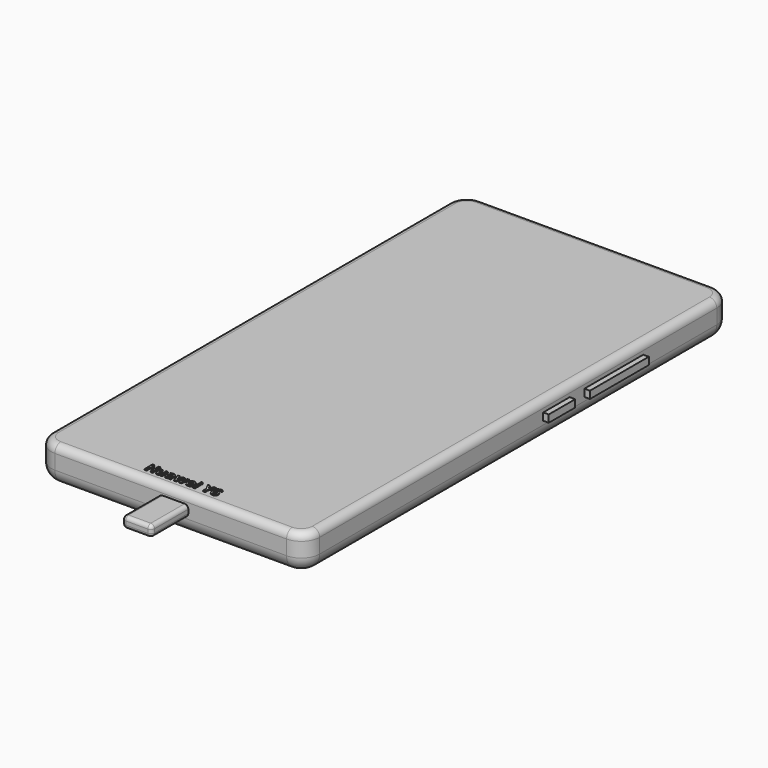
from build123d import *

# Parameters (mm, degrees)
F1_DEPTH      = 10
F2_R          = 2
F3_R          = 4
F4_W          = 20
F4_H          = 2
F5_DEPTH      = 38
F6_W          = 9
F6_H          = 2
F7_DEPTH      = 38
F8_W          = 8
F8_H          = 3
F9_DEPTH      = 85
F10_R         = 1
F11_TEXT_SIZE = 3.7978814942
F12_DEPTH     = 0.2


# Not quite as in the source:
# - Text() gives the source's letters only with a copy of the font that has no kerning and outlines rounded to 1/6400 em; it was checked with that copy


with BuildPart() as f1:
    # F0 (on Top) → F1 (new body)
    with BuildSketch(Plane.XY):
        with BuildLine():
            Line((-31.5, -72.5), (31.5, -72.5))
            ThreePointArc((31.5, -72.5), (35.0355339059, -71.0355339059), (36.5, -67.5))
            Line((36.5, -67.5), (36.5, 67.5))
            ThreePointArc((36.5, 67.5), (35.0355339059, 71.0355339059), (31.5, 72.5))
            Line((31.5, 72.5), (-31.5, 72.5))
            ThreePointArc((-31.5, 72.5), (-35.0355339059, 71.0355339059), (-36.5, 67.5))
            Line((-36.5, 67.5), (-36.5, -67.5))
            ThreePointArc((-36.5, -67.5), (-35.0355339059, -71.0355339059), (-31.5, -72.5))
        make_face()
    extrude(amount=F1_DEPTH)

    # F2
    f2_edges = [f1.edges().sort_by_distance(p)[0] for p in [
        (-35.035534, 71.035534, 10),
    ]]
    fillet(f2_edges, radius=F2_R)

    # F3
    f3_edges = [f1.edges().sort_by_distance(p)[0] for p in [
        (-35.035534, 71.035534, 0),
    ]]
    fillet(f3_edges, radius=F3_R)

    # F4 (on Right) → F5 (join)
    with BuildSketch(Plane.YZ):
        with Locations((32.5, 6)):
            Rectangle(F4_W, F4_H)
    extrude(amount=F5_DEPTH)

    # F6 (on Right) → F7 (join)
    with BuildSketch(Plane.YZ):
        with Locations((13, 6)):
            Rectangle(F6_W, F6_H)
    extrude(amount=F7_DEPTH)

    # F8 (on Front) → F9 (join)
    with BuildSketch(Plane.XZ):
        with Locations((0.7886027023, 5.945433151)):
            Rectangle(F8_W, F8_H)
    extrude(amount=F9_DEPTH)

    # F10
    f10_edges = [f1.edges().sort_by_distance(p)[0] for p in [
        (4.788603, -78.75, 7.445433),
        (0.788603, -85, 7.445433),
        (-3.211397, -78.75, 7.445433),
        (-3.211397, -85, 5.945433),
        (-3.211397, -78.75, 4.445433),
        (0.788603, -85, 4.445433),
        (4.788603, -78.75, 4.445433),
        (4.788603, -85, 5.945433),
    ]]
    fillet(f10_edges, radius=F10_R)

    # F11 (on face) → F12 (join)
    with BuildSketch(Plane.XY.offset(10)):
        with Locations((-9.8508823118, -69.5)):
            Text('Huawei Y6', F11_TEXT_SIZE, font='Open Sans', font_style=FontStyle.BOLD, text_align=(TextAlign.LEFT, TextAlign.BOTTOM))
    extrude(amount=F12_DEPTH)


solid = f1.part
